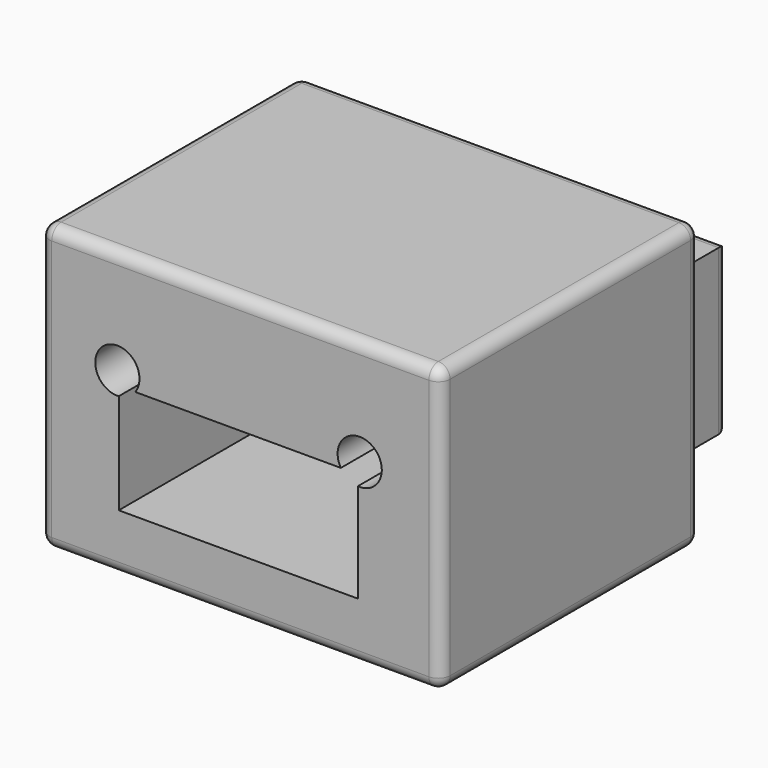
from build123d import *

# Parameters (mm, degrees)
F1_W          = 86.341727525
F1_H          = 61.3026246428
F2_DEPTH      = 69.85
F0_R          = 11.2874637249
F5_DEPTH      = 25.4
F6_DEPTH      = 6.35
F3_W          = 68.7855817378
F3_H          = 35.4001102969
F7_DEPTH      = 19.05
F8_R          = 2.54
F8_2_R        = 2.54
F9_T1_DEPTH   = 65.1126246428
F9_T3_DEPTH   = 90.151727525
F9_S7_W       = 2.54
F9_S7_H       = 2.54
F9_T8_DEPTH   = 2.54
F9_S13_W      = 2.54
F9_S13_H      = 2.54
F9_T14_DEPTH  = 2.54
F10_T1_DEPTH  = 64.77
F10_S5_W      = 2.54
F10_S5_H      = 2.54
F10_T6_DEPTH  = 2.54
F10_S11_W     = 2.54
F10_S11_H     = 2.54
F10_T12_DEPTH = 2.54
F11_R         = 4.7625
F12_DEPTH     = 279.4
F13_W         = 51.5172332525
F13_H         = 23.6000707373
F14_DEPTH     = 101.6


# Not quite as in the source:
# - a fillet or chamfer that OpenCascade refuses, or shapes differently, is made with other operations: its cross-section is extruded or revolved along the edge and cut away or added


with BuildPart() as f2:
    # F1 (on Front) → F2 (new body)
    with BuildSketch(Plane.XZ):
        with Locations((0.8634161204, 5.0365999341)):
            Rectangle(F1_W, F1_H)
    extrude(amount=F2_DEPTH)

    # F8
    f8_edges = [f2.edges().sort_by_distance(p)[0] for p in [
        (-42.307448, -34.925, 35.687912),
        (0.863416, 0, 35.687912),
        (44.03428, -34.925, 35.687912),
        (0.863416, -69.85, 35.687912),
        (44.03428, -69.85, 5.0366),
        (-42.307448, -69.85, 5.0366),
        (0.863416, -69.85, -25.614712),
        (44.03428, -34.925, -25.614712),
        (44.03428, 0, 5.0366),
    ]]
    fillet(f8_edges, radius=F8_R)

    # F9: fillet of radius 2.54 on 2 edges, made by hand

    # F9_s2 → F9_t1 (cut)
    with BuildSketch(Plane.XY.offset(-31.9647123873)):
        with BuildLine():
            ThreePointArc((-39.7674476421, 0), (-41.5634988663, -0.7439487758), (-42.3074476421, -2.54))
            Line((-42.3074476421, -2.54), (-42.3074476421, 0))
            Line((-42.3074476421, 0), (-39.7674476421, 0))
        make_face()
    extrude(amount=F9_T1_DEPTH, mode=Mode.SUBTRACT)

    # F9_s4 → F9_t3 (cut)
    with BuildSketch(Plane.YZ.offset(-48.6574476421)):
        with BuildLine():
            ThreePointArc((0, -23.0747123873), (-0.7439487758, -24.8707636115), (-2.54, -25.6147123873))
            Line((-2.54, -25.6147123873), (0, -25.6147123873))
            Line((0, -25.6147123873), (0, -23.0747123873))
        make_face()
    extrude(amount=F9_T3_DEPTH, mode=Mode.SUBTRACT)


with BuildPart() as f5:
    # F0 (on Front) → F5 (new body)
    with BuildSketch(Plane.XZ):
        with Locations((-13.1441846499, 0)):
            Circle(F0_R)
    extrude(amount=-F5_DEPTH)


with BuildPart() as f5b:
    # F0 (on Front) → F5, piece 2 (new body)
    with BuildSketch(Plane.XZ):
        with Locations((13.4262019347, 0)):
            Circle(F0_R)
    extrude(amount=-F5_DEPTH)


with BuildPart() as f6:
    # F4 (on Front) → F6 (new body)
    with BuildSketch(Plane.XZ):
        with BuildLine():
            add(Edge.make_bspline(
                [(33.0976620317, -7.1951444261), (31.1890209887, -3.2906266132), (19.0840525939, -3.2757250199), (27.6928798629, -53.6869881743), (36.5438211862, -14.2449717651), (33.0976620317, -7.1951444261)],
                knots=[0, 0, 0, 0, 0.2172144581, 0.6078070332, 1, 1, 1, 1], degree=3))
        make_face()
    extrude(amount=-F6_DEPTH)


with BuildPart() as f6b:
    # F4 (on Front) → F6, piece 2 (new body)
    with BuildSketch(Plane.XZ):
        with BuildLine():
            add(Edge.make_bspline(
                [(-23.7341076136, -7.1951444261), (-25.6427486565, -3.2906266132), (-37.7477170514, -3.2757250199), (-29.1388897823, -53.6869881743), (-20.287948459, -14.2449717651), (-23.7341076136, -7.1951444261)],
                knots=[0, 0, 0, 0, 0.2172144581, 0.6078070332, 1, 1, 1, 1], degree=3))
        make_face()
    extrude(amount=-F6_DEPTH)


with BuildPart() as f7:
    # F3 (on Front) → F7 (new body)
    with BuildSketch(Plane.XZ):
        with Locations((0.4317071289, 3.3097662963)):
            Rectangle(F3_W, F3_H)
    extrude(amount=-F7_DEPTH)

    # F8#2
    f8_2_edges = [f7.edges().sort_by_distance(p)[0] for p in [
        (0.431707, 19.05, 21.009821),
        (-33.961084, 19.05, 3.309766),
        (0.431707, 19.05, -14.390289),
        (34.824498, 19.05, 3.309766),
    ]]
    fillet(f8_2_edges, radius=F8_2_R)


with BuildPart() as f9_tool6:
    # F9_s7 → F9_t8 (new body)
    with BuildSketch(Plane.XZ.offset(2.54)):
        with Locations((42.7642798829, -24.3447123873)):
            Rectangle(F9_S7_W, F9_S7_H)
    extrude(amount=-F9_T8_DEPTH)

    # F9_s9 → F9_t10 (revolve, cut)
    with BuildSketch(Plane(origin=(41.4942798829, -2.54, -23.0747123873), x_dir=(-0.7071067812, 0, 0.7071067812), z_dir=(-0.7071067812, 0, -0.7071067812))):
        with BuildLine():
            ThreePointArc((0, -2.54), (2.54, 0), (0, 2.54))
            Line((0, 2.54), (0, -2.54))
        make_face()
    revolve(axis=Axis((41.4942798829, -2.54, -23.0747123873), (0, 1, 0)), mode=Mode.SUBTRACT)


with BuildPart() as f2_1:
    add(f2.part)

    # F9_t5: cut F9_tool6
    add(f9_tool6.part, mode=Mode.SUBTRACT)


with BuildPart() as f9_tool12:
    # F9_s13 → F9_t14 (new body)
    with BuildSketch(Plane.XZ.offset(2.54)):
        with Locations((-41.0374476421, 34.4179122555)):
            Rectangle(F9_S13_W, F9_S13_H)
    extrude(amount=-F9_T14_DEPTH)

    # F9_s15 → F9_t16 (revolve, cut)
    with BuildSketch(Plane(origin=(-39.7674476421, -2.54, 33.1479122555), x_dir=(0.7071067812, 0, -0.7071067812), z_dir=(0.7071067812, 0, 0.7071067812))):
        with BuildLine():
            ThreePointArc((0, -2.54), (2.54, 0), (0, 2.54))
            Line((0, 2.54), (0, -2.54))
        make_face()
    revolve(axis=Axis((-39.7674476421, -2.54, 33.1479122555), (0, 1, 0)), mode=Mode.SUBTRACT)


with BuildPart() as f2_2:
    add(f2_1.part)

    # F9_t11: cut F9_tool12
    add(f9_tool12.part, mode=Mode.SUBTRACT)

    # F10: fillet of radius 2.54 on 1 edges, made by hand

    # F10_s2 → F10_t1 (cut)
    with BuildSketch(Plane.XZ.offset(2.54)):
        with BuildLine():
            ThreePointArc((-39.7674476421, -25.6147123873), (-41.5634988663, -24.8707636115), (-42.3074476421, -23.0747123873))
            Line((-42.3074476421, -23.0747123873), (-42.3074476421, -25.6147123873))
            Line((-42.3074476421, -25.6147123873), (-39.7674476421, -25.6147123873))
        make_face()
    extrude(amount=F10_T1_DEPTH, mode=Mode.SUBTRACT)


with BuildPart() as f10_tool4:
    # F10_s5 → F10_t6 (new body)
    with BuildSketch(Plane.XY.offset(-23.0747123873)):
        with Locations((-41.0374476421, -1.27)):
            Rectangle(F10_S5_W, F10_S5_H)
    extrude(amount=-F10_T6_DEPTH)

    # F10_s7 → F10_t8 (revolve, cut)
    with BuildSketch(Plane(origin=(-39.7674476421, -2.54, -23.0747123873), x_dir=(0.7071067812, -0.7071067812, 0), z_dir=(0.7071067812, 0.7071067812, 0))):
        with BuildLine():
            ThreePointArc((0, -2.54), (2.54, 0), (0, 2.54))
            Line((0, 2.54), (0, -2.54))
        make_face()
    revolve(axis=Axis((-39.7674476421, -2.54, -23.0747123873), (0, 0, -1)), mode=Mode.SUBTRACT)


with BuildPart() as f2_3:
    add(f2_2.part)

    # F10_t3: cut F10_tool4
    add(f10_tool4.part, mode=Mode.SUBTRACT)


with BuildPart() as f10_tool10:
    # F10_s11 → F10_t12 (new body)
    with BuildSketch(Plane.XY.offset(-23.0747123873)):
        with Locations((-41.0374476421, -68.58)):
            Rectangle(F10_S11_W, F10_S11_H)
    extrude(amount=-F10_T12_DEPTH)

    # F10_s13 → F10_t14 (revolve, cut)
    with BuildSketch(Plane(origin=(-39.7674476421, -67.31, -23.0747123873), x_dir=(0.7071067812, 0.7071067812, 0), z_dir=(-0.7071067812, 0.7071067812, 0))):
        with BuildLine():
            ThreePointArc((0, -2.54), (2.54, 0), (0, 2.54))
            Line((0, 2.54), (0, -2.54))
        make_face()
    revolve(axis=Axis((-39.7674476421, -67.31, -23.0747123873), (0, 0, -1)), mode=Mode.SUBTRACT)


with BuildPart() as f2_4:
    add(f2_3.part)

    # F10_t9: cut F10_tool10
    add(f10_tool10.part, mode=Mode.SUBTRACT)


with BuildPart() as f12_tool:
    # F11 (on Front) → F12 (new body, symmetric)
    with BuildSketch(Plane.XZ):
        with Locations((26.5864427257, 12.8356372612)):
            Circle(F11_R)
        with Locations((-25.6259300993, 13.1550712943)):
            Circle(F11_R)
    extrude(amount=F12_DEPTH, both=True)


with BuildPart() as f2_5:
    add(f2_4.part)

    # F12: cut by f12_tool
    add(f12_tool.part, mode=Mode.SUBTRACT)

    # F13 (on Front) → F14 (cut)
    with BuildSketch(Plane.XZ):
        with Locations((0.4317108542, -1.4390288852)):
            Rectangle(F13_W, F13_H)
    extrude(amount=F14_DEPTH, mode=Mode.SUBTRACT)


with BuildPart() as f7_1:
    add(f7.part)

    # F12: cut by f12_tool
    add(f12_tool.part, mode=Mode.SUBTRACT)


solid = Compound([f5.part, f5b.part, f6.part, f6b.part, f2_5.part, f7_1.part])
